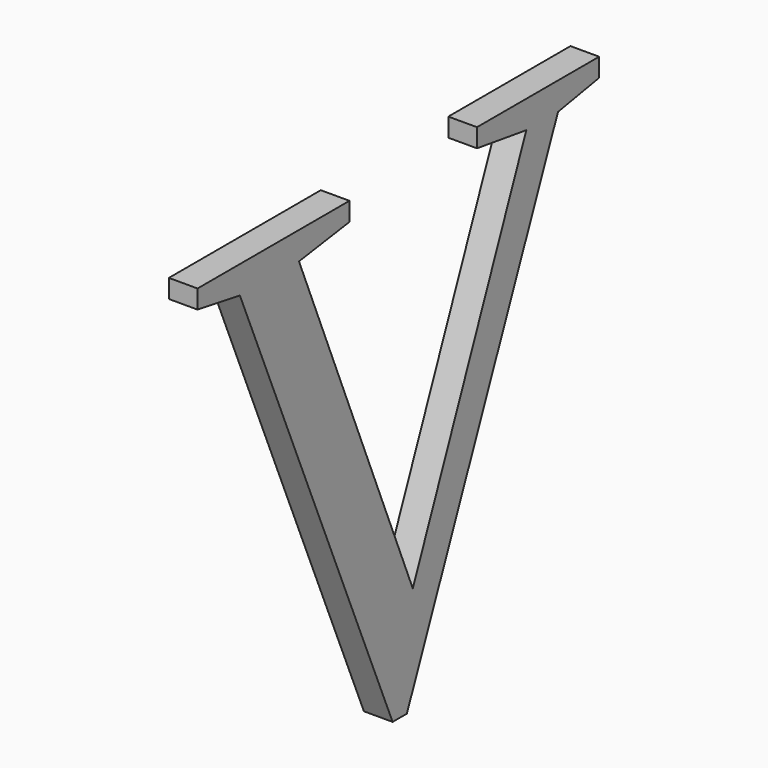
from build123d import *

# Parameters (mm, degrees)
F0_TEXT_SIZE = 635
F1_DEPTH     = 25.4


# Not quite as in the source:
# - Text() gives the source's letters only with a copy of the font that has no kerning and outlines rounded to 1/6400 em; it was checked with that copy


with BuildPart() as f1:
    # F0 (on Right) → F1 (new body)
    with BuildSketch(Plane.YZ):
        with Locations((-451.4453125, 0)):
            Text('V', F0_TEXT_SIZE, font='Tinos', text_align=(TextAlign.LEFT, TextAlign.BOTTOM))
    extrude(amount=F1_DEPTH)


solid = f1.part
